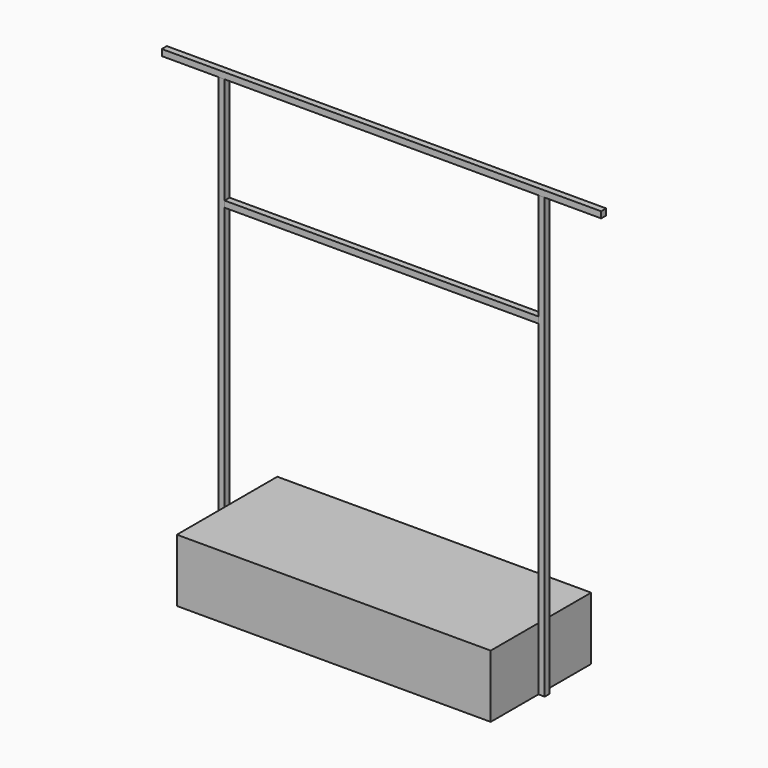
from build123d import *

# Parameters (mm, degrees)
F1_DEPTH  = 250
F3_DEPTH  = 714
F5_DEPTH  = 625
F7_DEPTH  = 608
F9_DEPTH  = 250
F11_DEPTH = 534
F15_W     = 25
F15_H     = 1750
F16_DEPTH = 12.5
F17_W     = 1750
F17_H     = 25
F18_DEPTH = 12.5
F19_W     = 25
F19_H     = 25
F20_DEPTH = 1250
F21_R     = 2.5
F22_DEPTH = 638
F23_R     = 2.5
F24_DEPTH = 639.7


with BuildPart() as f1:
    # F0 (on Front) → F1 (new body, symmetric)
    with BuildSketch(Plane.XZ):
        Polygon((-607, 18), (-625, 0), (625, 0), (607, 18), align=None)
    extrude(amount=F1_DEPTH, both=True)

    # F2 (on Right) → F3 (cut, symmetric)
    with BuildSketch(Plane.YZ):
        Polygon((-266.0376429558, 0), (-250, 0), (-231.0939141602, 18.9060858398), (-231.0939141602, 28.4129753709), (-266.0376429558, 28.4129753709), align=None)
        Polygon((231.0939141602, 18.9060858398), (250, 0), (262.9185318947, 0), (262.9185318947, 44.0045437723), (231.0939141602, 44.0045437723), align=None)
    extrude(amount=F3_DEPTH, both=True, mode=Mode.SUBTRACT)


with BuildPart() as f5:
    # F4 (on Right) → F5 (new body, symmetric)
    with BuildSketch(Plane.YZ):
        Polygon((232, 232), (232, 18), (250, 0), (250, 250), align=None)
    extrude(amount=F5_DEPTH, both=True)


with BuildPart() as f5b:
    # F4 (on Right) → F5, piece 2 (new body, symmetric)
    with BuildSketch(Plane.YZ):
        Polygon((-250, 0), (-232, 18), (-232, 232), (-250, 250), align=None)
    extrude(amount=F5_DEPTH, both=True)


with BuildPart() as f7_tool:
    # F6 (on Top) → F7 (new body, symmetric)
    with BuildSketch(Plane.XY):
        Polygon((-607, 232), (-625, 250), (-625, 212.7924200636), (-607, 212.7924200636), align=None)
        Polygon((-625, -250), (-607, -232), (-638.8453841209, -232), (-638.8453841209, -250), align=None)
        Polygon((625, 212.7924200636), (625, 250), (607, 232), (607, 212.7924200636), align=None)
        Polygon((638.8453841209, -250), (638.8453841209, -232), (607, -232), (625, -250), align=None)
    extrude(amount=F7_DEPTH, both=True)


with BuildPart() as f5_1:
    add(f5.part)

    # F7: cut by f7_tool
    add(f7_tool.part, mode=Mode.SUBTRACT)


with BuildPart() as f5b_1:
    add(f5b.part)

    # F7: cut by f7_tool
    add(f7_tool.part, mode=Mode.SUBTRACT)


with BuildPart() as f9:
    # F8 (on Front) → F9 (new body, symmetric)
    with BuildSketch(Plane.XZ):
        Polygon((-625, 250), (-625, 0), (-607, 18), (-607, 232), align=None)
    extrude(amount=F9_DEPTH, both=True)

    # F10 (on Top) → F11 (cut, symmetric)
    with BuildSketch(Plane.XY):
        Polygon((-596.8062881455, -232), (-607, -232), (-625, -250), (-625, -280.7182726889), (-596.8062881455, -280.7182726889), align=None)
        Polygon((-625, 250), (-607, 232), (-596.8062881455, 234.6027734251), (-596.8062881455, 288.4899377823), (-625, 288.4899377823), align=None)
    extrude(amount=F11_DEPTH, both=True, mode=Mode.SUBTRACT)


with BuildPart() as f12_1:
    # F12: instance of F9
    add(f9.part.mirror(Plane.YZ))


with BuildPart() as f14_1:
    # F14: instance of F1
    add(f1.part.mirror(Plane.XY.offset(125)))


with BuildPart() as f16:
    # F15 (on Front) → F16 (new body, symmetric)
    with BuildSketch(Plane.XZ):
        with Locations((637.5, 875)):
            Rectangle(F15_W, F15_H)
    extrude(amount=F16_DEPTH, both=True)


with BuildPart() as f16b:
    # F15 (on Front) → F16, piece 2 (new body, symmetric)
    with BuildSketch(Plane.XZ):
        with Locations((-637.5, 875)):
            Rectangle(F15_W, F15_H)
    extrude(amount=F16_DEPTH, both=True)


with BuildPart() as f18:
    # F17 (on Front) → F18 (new body, symmetric)
    with BuildSketch(Plane.XZ):
        with Locations((0, 1762.5)):
            Rectangle(F17_W, F17_H)
    extrude(amount=F18_DEPTH, both=True)


with BuildPart() as f20:
    # F19 (on face) → F20 (new body, through all)
    with BuildSketch(Plane.YZ.offset(-625)):
        with Locations((0, 1312.5)):
            Rectangle(F19_W, F19_H)
    extrude(amount=F20_DEPTH)


with BuildPart() as f22_tool:
    # F21 (on Right) → F22 (new body, symmetric)
    with BuildSketch(Plane.YZ):
        with Locations((0, 180)):
            Circle(F21_R)
        with Locations((0, 70)):
            Circle(F21_R)
    extrude(amount=F22_DEPTH, both=True)


with BuildPart() as f16_1:
    add(f16.part)

    # F22: cut by f22_tool
    add(f22_tool.part, mode=Mode.SUBTRACT)


with BuildPart() as f16b_1:
    add(f16b.part)

    # F22: cut by f22_tool
    add(f22_tool.part, mode=Mode.SUBTRACT)


with BuildPart() as f24_tool:
    # F23 (on Right) → F24 (new body, symmetric)
    with BuildSketch(Plane.YZ):
        with Locations((0, 1312.5)):
            Circle(F23_R)
    extrude(amount=F24_DEPTH, both=True)


with BuildPart() as f16_2:
    add(f16_1.part)

    # F24: cut by f24_tool
    add(f24_tool.part, mode=Mode.SUBTRACT)


with BuildPart() as f16b_2:
    add(f16b_1.part)

    # F24: cut by f24_tool
    add(f24_tool.part, mode=Mode.SUBTRACT)


solid = Compound([f1.part, f5_1.part, f5b_1.part, f9.part, f12_1.part, f14_1.part, f18.part, f20.part, f16_2.part, f16b_2.part])
